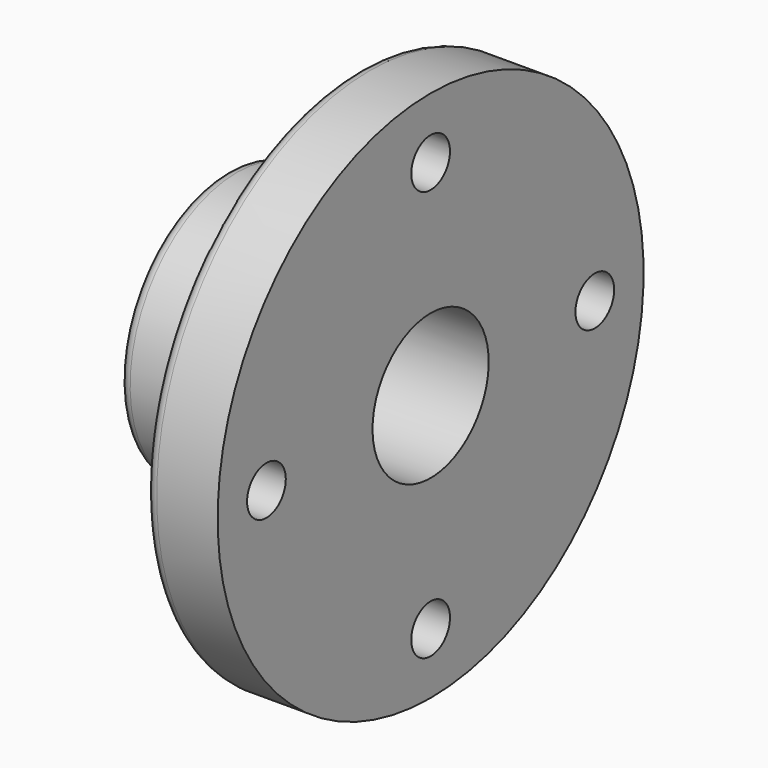
from build123d import *

# Parameters (mm, degrees)
F2_R            = 6.35
F3_DEPTH        = 19.051
F3_COPIES_COUNT = 4
F4_R            = 3.048


# Not quite as in the source:
# - a pattern or mirror of a feature is missing from the dataset's text; its kind, count and spacing are read off the source's solid


with BuildPart() as f1:
    # F0 (on Front) → F1 (revolve)
    with BuildSketch(Plane.XZ):
        Polygon((0, 35.052), (0, 19.05), (53.848, 19.05), (53.848, 69.85), (34.798, 69.85), (34.798, 35.052), align=None)
    revolve(axis=Axis((26.924, 0, 0), (1, 0, 0)))

    # F2 (on face) → F3 (cut, through all)
    with BuildSketch(Plane(origin=(34.798, 0, 0), x_dir=(0, -1, 0), z_dir=(-1, 0, 0))):
        with Locations((0, 53.848)):
            Circle(F2_R)
    f3 = extrude(amount=-F3_DEPTH, mode=Mode.SUBTRACT)

    # F3_copies: F3 ×4 about axis
    f3_copies_axis = Axis((0, 0, 0), (1, 0, 0))
    for i in range(1, F3_COPIES_COUNT):
        add(f3.rotate(f3_copies_axis, i * 360 / F3_COPIES_COUNT), mode=Mode.SUBTRACT)

    # F4
    f4_edges = [f1.edges().sort_by_distance(p)[0] for p in [
        (0, 0, -35.052),
        (34.798, 0, -69.85),
    ]]
    fillet(f4_edges, radius=F4_R)


solid = f1.part
